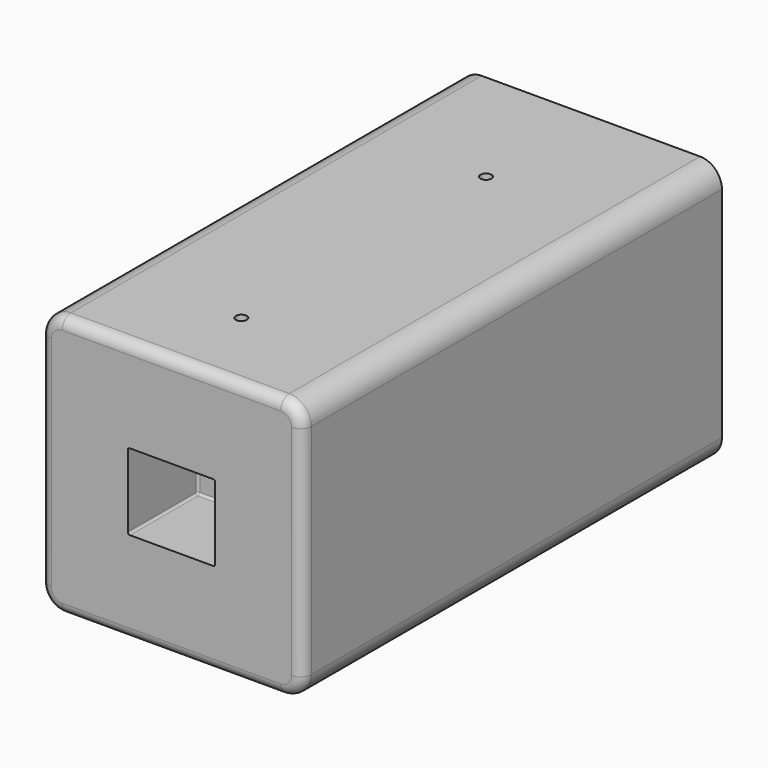
from build123d import *

# Parameters (mm, degrees)
F0_W     = 304.8
F0_H     = 304.8
F0_W_2   = 101.6
F0_H_2   = 88.9
F1_DEPTH = 609.6
F8_DEPTH = 508
F2_R     = 25.4
F3_R     = 12.7
F4_D     = 12.7
F4_DEPTH = 38.1
F4_TIP   = 3.8154649308
F6_D     = 12.7
F6_DEPTH = 38.1
F6_TIP   = 3.8154649308
F7_R     = 2.54


# Not quite as in the source:
# - a feature names something its author has since deleted; it is built from what else it names


with BuildPart() as f1:
    # F0 (on Front) → F1 (new body)
    with BuildSketch(Plane.XZ):
        Rectangle(F0_W, F0_H)
        Rectangle(F0_W_2, F0_H_2, mode=Mode.SUBTRACT)
    extrude(amount=F1_DEPTH)

    # F0 (on Front) → F8 (join)
    with BuildSketch(Plane.XZ):
        Rectangle(F0_W_2, F0_H_2)
    extrude(amount=F8_DEPTH)

    # F2
    f2_edges = [f1.edges().sort_by_distance(p)[0] for p in [
        (152.4, -304.8, -152.4),
        (-152.4, -304.8, -152.4),
        (-152.4, -304.8, 152.4),
        (152.4, -304.8, 152.4),
    ]]
    fillet(f2_edges, radius=F2_R)

    # F3
    f3_edges = [f1.edges().sort_by_distance(p)[0] for p in [
        (152.4, -609.6, 0),
    ]]
    fillet(f3_edges, radius=F3_R)

    # F4
    with Locations(Plane(origin=(0, 0, -152.4), x_dir=(1, 0, 0), z_dir=(0, 0, -1))):
        with Locations((0, 152.4), (0, 508)):
            Hole(F4_D / 2, depth=F4_DEPTH)
            with Locations((0, 0, -(F4_DEPTH + F4_TIP / 2))):  # 118° drill point
                Cone(0, F4_D / 2, F4_TIP, mode=Mode.SUBTRACT)

    # F6
    with Locations(Plane.XY.offset(152.4)):
        with Locations((0, -508), (0, -152.4)):
            Hole(F6_D / 2, depth=F6_DEPTH)
            with Locations((0, 0, -(F6_DEPTH + F6_TIP / 2))):  # 118° drill point
                Cone(0, F6_D / 2, F6_TIP, mode=Mode.SUBTRACT)

    # F7
    f7_edges = [f1.edges().sort_by_distance(p)[0] for p in [
        (-50.8, -558.8, -44.45),
        (-50.8, -558.8, 44.45),
        (50.8, -558.8, 44.45),
        (50.8, -558.8, -44.45),
        (50.8, -508, 0),
        (0, -508, 44.45),
        (-50.8, -508, 0),
        (0, -508, -44.45),
    ]]
    fillet(f7_edges, radius=F7_R)


solid = f1.part
